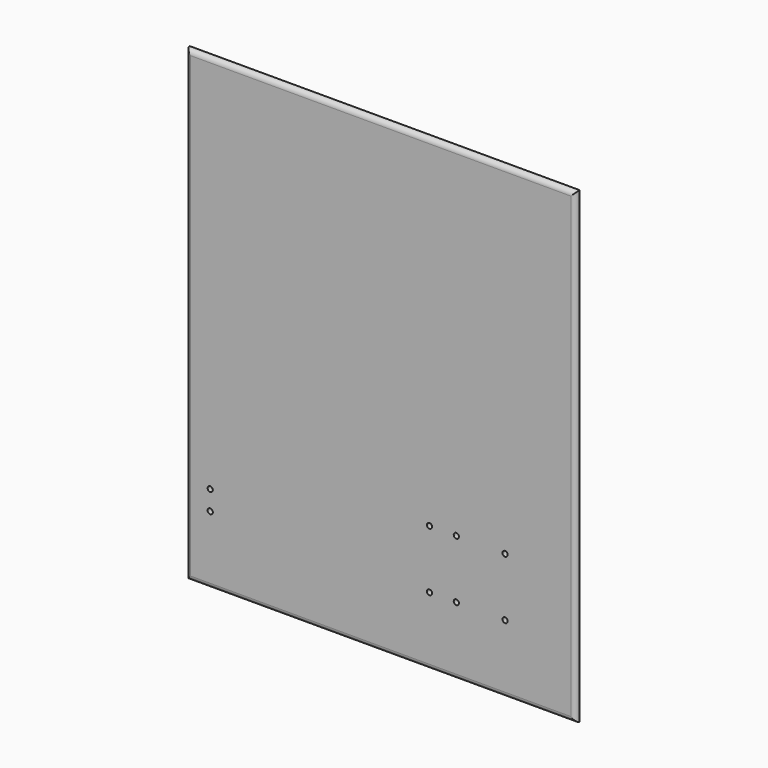
from build123d import *

# Parameters (mm, degrees)
F1_DEPTH = 6.35
F2_R     = 6.34999
F3_D     = 6.7564


# Not quite as in the source:
# - a fillet or chamfer is up to 0.001 mm smaller than in the source, because OpenCascade refuses the exact size


with BuildPart() as f1:
    # F0 (on Front) → F1 (new body)
    with BuildSketch(Plane.XZ):
        Polygon((-494.6137029603, 259.7943879247), (-494.6137029603, -45.0056120753), (13.3862970397, -45.0056120753), (13.3862970397, 259.7943879247), (13.3862970397, 564.5943879247), (-494.6137029603, 564.5943879247), align=None)
    extrude(amount=F1_DEPTH)

    # F2 (radius 6.35 in the source; OpenCascade refuses exactly that, so slightly less here)
    f2_edges = [f1.edges().sort_by_distance(p)[0] for p in [
        (-494.613703, -6.35, 259.794388),
        (-240.613703, -6.35, -45.005612),
        (13.386297, -6.35, 259.794388),
        (-240.613703, -6.35, 564.594388),
    ]]
    fillet(f2_edges, radius=F2_R)

    # F3 (through all)
    with Locations(Plane(origin=(0, 0, 0), x_dir=(1, 0, 0), z_dir=(0, 1, 0))):
        with Locations((-177.1137029603, -120.0943879247), (-142.1887029603, -120.0943879247), (-78.6887029603, -120.0943879247), (-78.6887029603, -43.8943879247), (-142.1887029603, -43.8943879247), (-177.1137029603, -43.8943879247), (-462.8637029603, -69.2943879247), (-462.8637029603, -43.8943879247)):
            Hole(F3_D / 2)


solid = f1.part
